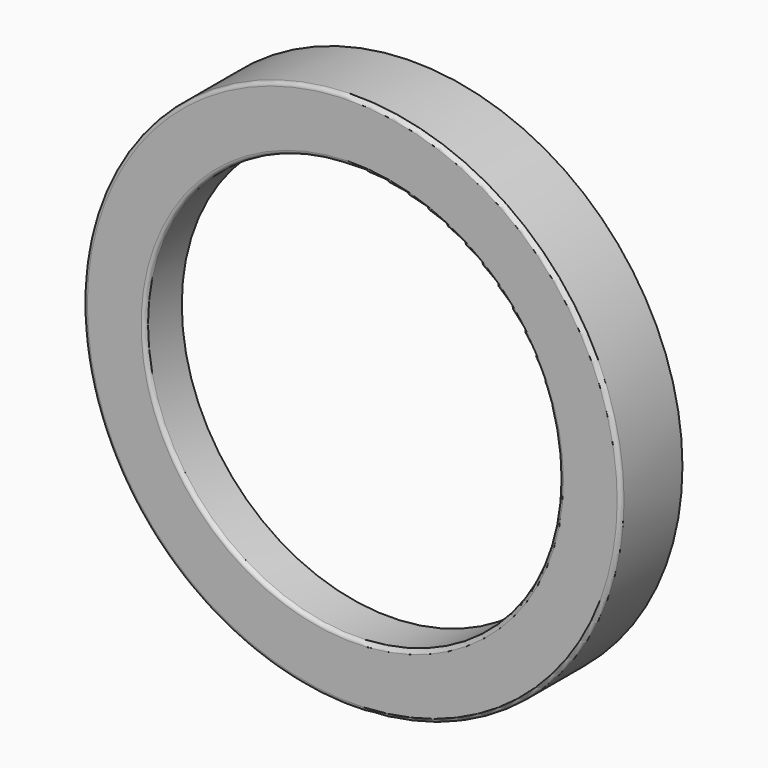
from build123d import *

# Parameters (mm, degrees)
F0_R     = 17.5
F0_R_2   = 13.5
F1_DEPTH = 5
F2_R     = 0.25
F3_R     = 16
F4_DEPTH = 2
F5_R     = 1.99999


# Not quite as in the source:
# - a fillet or chamfer is up to 0.001 mm smaller than in the source, because OpenCascade refuses the exact size


with BuildPart() as f1:
    # F0 (on Front) → F1 (new body)
    with BuildSketch(Plane.XZ):
        Circle(F0_R)
        Circle(F0_R_2, mode=Mode.SUBTRACT)
    extrude(amount=F1_DEPTH)

    # F2
    f2_edges = [f1.edges().sort_by_distance(p)[0] for p in [
        (-17.5, -5, 0),
        (-13.5, -5, 0),
    ]]
    fillet(f2_edges, radius=F2_R)

    # F3 (on Front) → F4 (cut)
    with BuildSketch(Plane.XZ):
        Circle(F3_R)
    extrude(amount=F4_DEPTH, mode=Mode.SUBTRACT)

    # F5 (radius 2 in the source; OpenCascade refuses exactly that, so slightly less here)
    f5_edges = [f1.edges().sort_by_distance(p)[0] for p in [
        (-16, -2, 0),
    ]]
    fillet(f5_edges, radius=F5_R)


solid = f1.part
